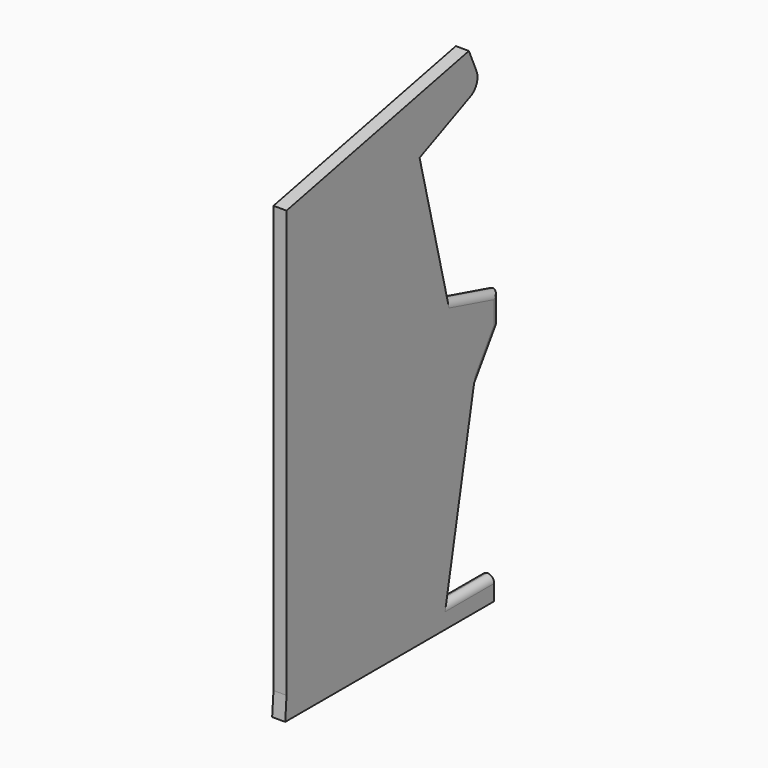
from build123d import *

# Parameters (mm, degrees)
F1_DEPTH     = 3.81
F2_R         = 4.2924717139
F3_R         = 2.032
F4_T4_DEPTH  = 27.583079529
F5_R         = 2.032
F6_T1_DEPTH  = 18.831700203
F6_T6_DEPTH  = 29.7046687957
F6_T11_DEPTH = 27.9890917976


# Not quite as in the source:
# - a fillet or chamfer that OpenCascade refuses, or shapes differently, is made with other operations: its cross-section is extruded or revolved along the edge and cut away or added


with BuildPart() as f1:
    # F0 (on Right) → F1 (new body)
    with BuildSketch(Plane.YZ):
        Polygon((-48.4873987734, 60.7866533101), (-48.4873987734, 33.8229238987), (-48.4873987734, 28.1463507563), (-48.4873987734, -63.624933362), (-48.9604510367, -70.247605443), (27.200255543, -70.247605443), (27.200255543, -63.624933362), (9.6974885091, -63.624933362), (19.158443436, -14.901005663), (29.0924459696, 0), (29.0924459696, 8.7513877079), (10.1705361158, 13.954914175), (0, 54.6370334923), (22.4697776139, 64.5710304379), (17.9654553963, 74.7593885665), align=None)
    extrude(amount=F1_DEPTH)

    # F2
    f2_edges = [f1.edges().sort_by_distance(p)[0] for p in [
        (1.905, 22.469778, 64.57103),
    ]]
    fillet(f2_edges, radius=F2_R)

    # F3
    f3_edges = [f1.edges().sort_by_distance(p)[0] for p in [
        (3.81, 18.448872, -63.624933),
    ]]
    fillet(f3_edges, radius=F3_R)

    # F4: fillet of radius 2.032 on 1 edges, made by hand


with BuildPart() as f4_tool2:
    # F4_s3 → F4_t4 (new body)
    with BuildSketch(Plane.XZ.offset(-32.2404117906)):
        with BuildLine():
            ThreePointArc((1.778, -63.624933362), (0.508, -64.296954195), (0, -65.640995861))
            Line((0, -65.640995861), (0, -63.624933362))
            Line((0, -63.624933362), (1.778, -63.624933362))
        make_face()
    extrude(amount=F4_T4_DEPTH)

    split(bisect_by=Plane(origin=(0, 21.2506127093, -4.1263317328), x_dir=(1, 0, 0), z_dir=(0, 0.981664966, -0.1906145181)), keep=Keep.TOP)


with BuildPart() as f1_1:
    add(f1.part)

    # F4_t1: cut F4_tool2
    add(f4_tool2.part, mode=Mode.SUBTRACT)

    # F5
    f5_edges = [f1_1.edges().sort_by_distance(p)[0] for p in [
        (0, 24.125445, -7.450503),
        (0, 29.092446, 4.375694),
        (0, 19.631491, 11.353151),
    ]]
    fillet(f5_edges, radius=F5_R)

    # F6: fillet of radius 2.032 on 3 edges, made by hand

    # F6_s2 → F6_t1 (cut)
    with BuildSketch(Plane.XY.offset(-5.0401562476)):
        with BuildLine():
            ThreePointArc((3.81, 27.0763834706), (3.302, 28.4204251366), (2.032, 29.0924459696))
            Line((2.032, 29.0924459696), (2.03708, 29.1327672196))
            ThreePointArc((2.03708, 29.1327672196), (2.921, 29.1330859696), (3.81, 29.1330859696))
            Line((3.81, 29.1330859696), (3.85064, 29.0924459696))
            Line((3.85064, 29.0924459696), (3.85064, 27.0763834706))
            Line((3.85064, 27.0763834706), (3.81, 27.0763834706))
        make_face()
    extrude(amount=F6_T1_DEPTH, mode=Mode.SUBTRACT)


with BuildPart() as f6_tool4:
    # F6_s5 → F6_t6 (new body)
    with BuildSketch(Plane(origin=(0, 29.6693335374, -8.1590686942), x_dir=(1, 0, 0), z_dir=(0, -0.9642053764, 0.2651565426))):
        with BuildLine():
            ThreePointArc((3.81, 14.1361249687), (3.302, 15.4801666347), (2.032, 16.1521874677))
            Line((2.032, 16.1521874677), (2.03708, 16.1925087177))
            ThreePointArc((2.03708, 16.1925087177), (2.921, 16.1928274677), (3.81, 16.1928274677))
            Line((3.81, 16.1928274677), (3.85064, 16.1521874677))
            Line((3.85064, 16.1521874677), (3.85064, 14.1361249687))
            Line((3.85064, 14.1361249687), (3.81, 14.1361249687))
        make_face()
    extrude(amount=F6_T6_DEPTH)

    split(bisect_by=Plane(origin=(0, 12.8557795978, 3.213946886), x_dir=(1, 0, 0), z_dir=(0, 0.9701424649, 0.2425357661)), keep=Keep.TOP)


with BuildPart() as f1_2:
    add(f1_1.part)

    # F6_t3: cut F6_tool4
    add(f6_tool4.part, mode=Mode.SUBTRACT)


with BuildPart() as f6_tool9:
    # F6_s10 → F6_t11 (new body)
    with BuildSketch(Plane(origin=(0, -3.7782576637, -5.6673872039), x_dir=(1, 0, 0), z_dir=(0, 0.5547001482, 0.8320503263))):
        with BuildLine():
            ThreePointArc((2.032, 24.206379163), (3.302, 23.53435833), (3.81, 22.190316664))
            Line((3.81, 22.190316664), (3.85064, 22.190316664))
            Line((3.85064, 22.190316664), (3.85064, 24.206379163))
            Line((3.85064, 24.206379163), (3.81, 24.247019163))
            ThreePointArc((3.81, 24.247019163), (2.921, 24.247019163), (2.03708, 24.246700413))
            Line((2.03708, 24.246700413), (2.032, 24.206379163))
        make_face()
    extrude(amount=F6_T11_DEPTH)

    split(bisect_by=Plane(origin=(0, 21.2506127093, -4.1263317328), x_dir=(1, 0, 0), z_dir=(0, 0.981664966, -0.1906145181)), keep=Keep.TOP)


with BuildPart() as f1_3:
    add(f1_2.part)

    # F6_t8: cut F6_tool9
    add(f6_tool9.part, mode=Mode.SUBTRACT)


solid = f1_3.part
